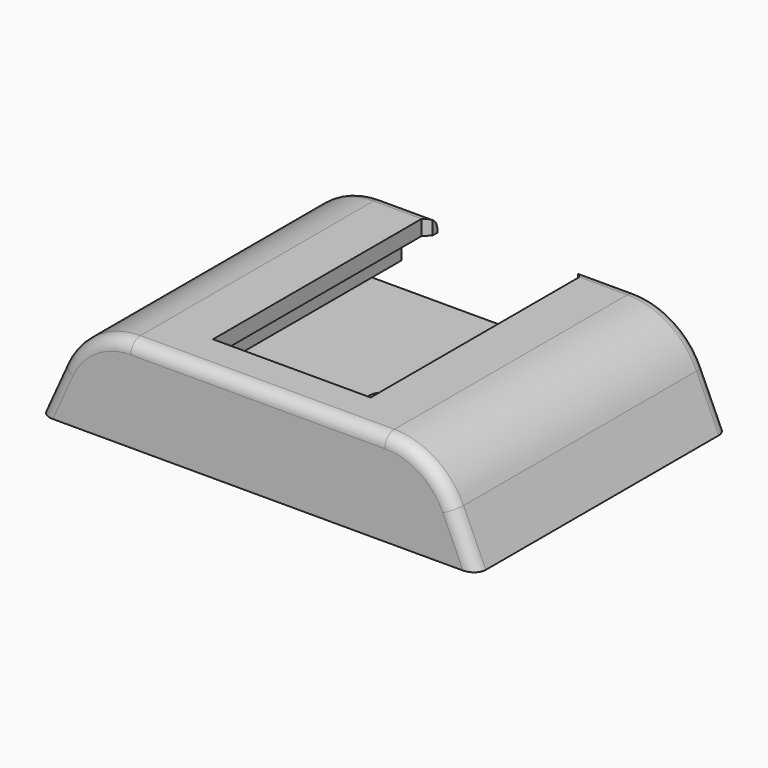
from build123d import *

# Parameters (mm, degrees)
F1_DEPTH  = 20
F3_DEPTH  = 2
F0_W      = 0.4
F0_H      = 1
F4_DEPTH  = 0.8
F5_SIZE   = 0.39999
F6_R      = 5
F7_R      = 0.79999
F8_SIZE   = 1
F9_R      = 1
F10_DEPTH = 1.2


# Not quite as in the source:
# - a fillet or chamfer is up to 0.001 mm smaller than in the source, because OpenCascade refuses the exact size


with BuildPart() as f1:
    # F0 (on Front) → F1 (new body)
    with BuildSketch(Plane.XZ):
        Polygon((9.6, -5), (0, -5), (-9.6, -5), (-9.6, -2.7), (-6.35, -2.7), (-6.35, -1), (-5.2, -1), (-5.2, 0), (-11.6, 0), (-14.4, -6.2), (0, -6.2), (14.4, -6.2), (11.6, 0), (5.2, 0), (5.2, -1), (6.35, -1), (6.35, -2.7), (9.6, -2.7), align=None)
    extrude(amount=F1_DEPTH)

    # F2 (on face) → F3 (join)
    with BuildSketch(Plane.XZ.offset(20)):
        Polygon((-5.2, 0), (-11.6, 0), (-14.4, -6.2), (11.6, -6.2), (11.6, 0), (5.2, 0), (5.2, -1), (6.35, -1), (6.35, -2.7), (9.6, -2.7), (9.6, -5), (-9.6, -5), (-9.6, -2.7), (-6.35, -2.7), (-6.35, -1), (-5.2, -1), align=None)
        Polygon((5.2, 0), (-5.2, 0), (-5.2, -1), (-6.35, -1), (-6.35, -2.7), (-9.6, -2.7), (-9.6, -5), (9.6, -5), (9.6, -2.7), (6.35, -2.7), (6.35, -1), (5.2, -1), align=None)
    extrude(amount=-F3_DEPTH)

    # F0 (on Front) + F3_face (on face) + F3_face1 (on face) → F4 (join)
    with BuildSketch(Plane.XZ):
        with Locations((5, -0.5)):
            Rectangle(F0_W, F0_H)
        with Locations((-5, -0.5)):
            Rectangle(F0_W, F0_H)
    with BuildSketch(Plane(origin=(0, -18, -2.8254432042), x_dir=(1, 0, 0), z_dir=(0, 1, 0))):
        Polygon((-5.2, -2.8254432042), (5.2, -2.8254432042), (5.2, -1.8254432042), (6.35, -1.8254432042), (6.35, -0.1254432042), (9.6, -0.1254432042), (9.6, 2.1745567958), (-9.6, 2.1745567958), (-9.6, -0.1254432042), (-6.35, -0.1254432042), (-6.35, -1.8254432042), (-5.2, -1.8254432042), align=None)
    with BuildSketch(Plane(origin=(0, -20, -3.2112820513), x_dir=(1, 0, 0), z_dir=(0, -1, 0))):
        Polygon((14.4, -2.9887179487), (11.6, 3.2112820513), (-11.6, 3.2112820513), (-14.4, -2.9887179487), align=None)
    extrude(amount=F4_DEPTH, dir=(0, -1, 0))

    # F5 (size 0.4 in the source; OpenCascade refuses exactly that, so slightly less here)
    f5_edges = [f1.edges().sort_by_distance(p)[0] for p in [
        (-4.8, -0.8, -0.5),
        (4.8, -0.8, -0.5),
    ]]
    chamfer(f5_edges, length=F5_SIZE)

    # F6
    f6_edges = [f1.edges().sort_by_distance(p)[0] for p in [
        (11.6, -10.4, 0),
        (-11.6, -10.4, 0),
    ]]
    fillet(f6_edges, radius=F6_R)

    # F7 (radius 0.8 in the source; OpenCascade refuses exactly that, so slightly less here)
    f7_edges = [f1.edges().sort_by_distance(p)[0] for p in [
        (13.664338, -20.8, -4.571033),
        (13.664338, 0, -4.571033),
        (-11.083863, 0, -0.799425),
    ]]
    fillet(f7_edges, radius=F7_R)

    # F8
    f8_edges = [f1.edges().sort_by_distance(p)[0] for p in [
        (-9.6, 0, -3.85),
        (-6.35, 0, -1.85),
        (6.35, 0, -1.85),
        (9.6, 0, -3.85),
    ]]
    chamfer(f8_edges, length=F8_SIZE)

    # F9 (on face) → F10 (cut, through all)
    with BuildSketch(Plane(origin=(0, 0, -6.2), x_dir=(1, 0, 0), z_dir=(0, 0, -1))):
        with Locations((0, 10.4)):
            Circle(F9_R)
    extrude(amount=-F10_DEPTH, mode=Mode.SUBTRACT)


solid = f1.part
